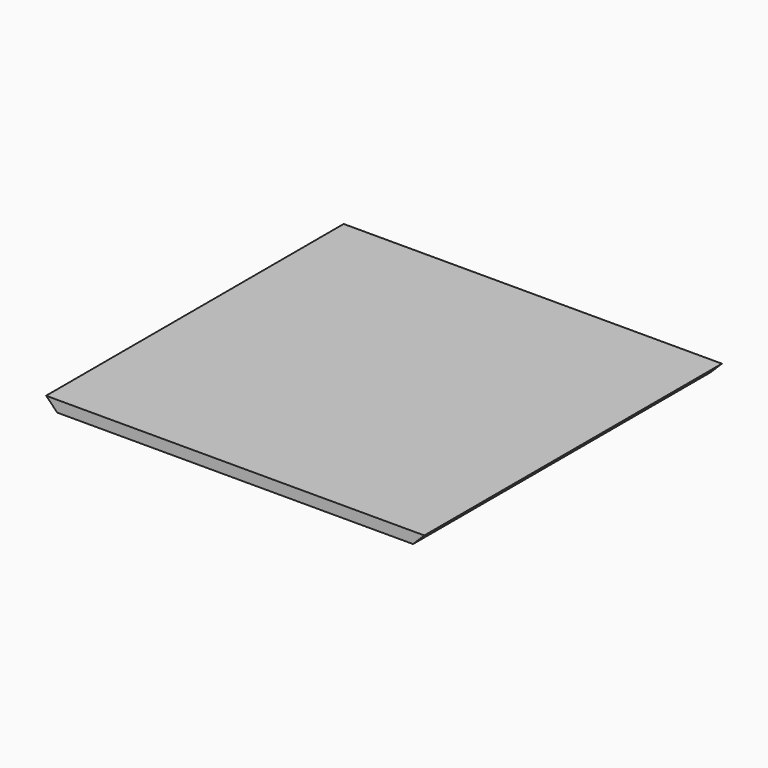
from build123d import *

# Parameters (mm, degrees)
F0_W     = 605
F0_H     = 595
F1_DEPTH = 18
F2_SIZE  = 17.99999


# Not quite as in the source:
# - a fillet or chamfer is up to 0.001 mm smaller than in the source, because OpenCascade refuses the exact size


with BuildPart() as f1:
    # F0 (on Top) → F1 (new body)
    with BuildSketch(Plane.XY):
        with Locations((2.1061599255, 30.7130831559)):
            Rectangle(F0_W, F0_H)
    extrude(amount=-F1_DEPTH)

    # F2 (size 18 in the source; OpenCascade refuses exactly that, so slightly less here)
    f2_edges = [f1.edges().sort_by_distance(p)[0] for p in [
        (-300.39384, 30.713083, -18),
        (304.60616, 30.713083, -18),
    ]]
    chamfer(f2_edges, length=F2_SIZE)


solid = f1.part
